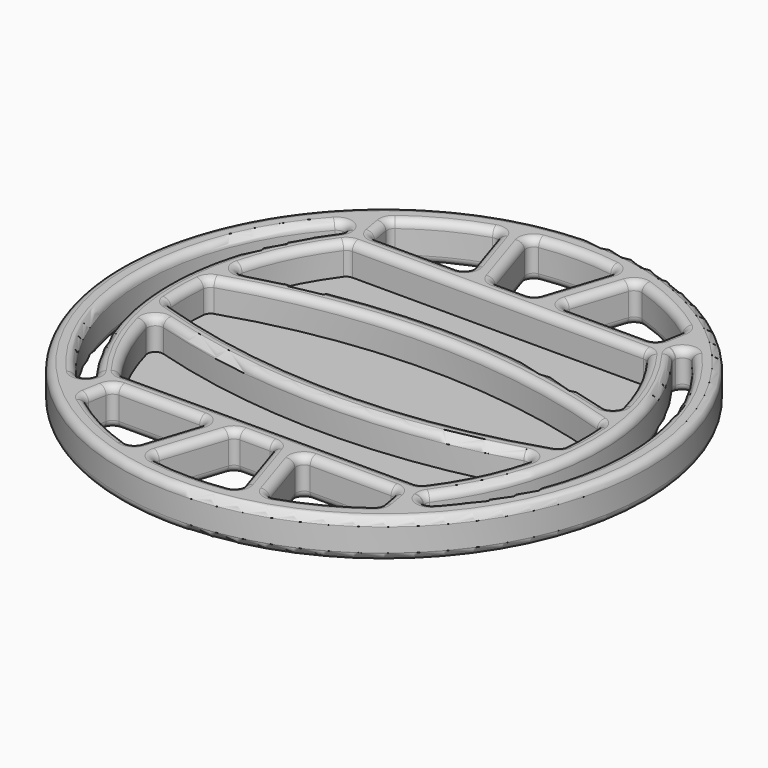
from build123d import *

# Parameters (mm, degrees)
F0_R     = 27.5
F1_DEPTH = 4
F2_DEPTH = 0.8
F3_F1_R  = 0.8
F3_F2_R  = 0.8
F3_F3_R  = 0.8


with BuildPart() as f1:
    # F0 (on Top) → F1 (new body)
    with BuildSketch(Plane.XY):
        Circle(F0_R)
        with BuildLine():
            ThreePointArc((17.4992602404, 17.994051546), (23.1218666205, 9.7667437759), (25.1, 0))
            ThreePointArc((25.1, 0), (23.1218666205, -9.7667437759), (17.4992602404, -17.994051546))
            ThreePointArc((17.4992602404, -17.994051546), (16.4683535979, -18.9421046818), (15.3861717662, -19.8311804586))
            ThreePointArc((15.3861717662, -19.8311804586), (11.4042701214, -22.359620368), (7.0196312763, -24.098439301))
            ThreePointArc((7.0196312763, -24.098439301), (5.8558617583, -24.4073530533), (4.6786166552, -24.6601002876))
            ThreePointArc((4.6786166552, -24.6601002876), (0, -25.1), (-4.6786166552, -24.6601002876))
            ThreePointArc((-4.6786166552, -24.6601002876), (-5.8558617583, -24.4073530533), (-7.0196312763, -24.098439301))
            ThreePointArc((-7.0196312763, -24.098439301), (-11.4042701214, -22.359620368), (-15.3861717662, -19.8311804586))
            ThreePointArc((-15.3861717662, -19.8311804586), (-16.4683535979, -18.9421046818), (-17.4992602404, -17.994051546))
            ThreePointArc((-17.4992602404, -17.994051546), (-25.1, 0), (-17.4992602404, 17.994051546))
            ThreePointArc((-17.4992602404, 17.994051546), (-16.4683535979, 18.9421046818), (-15.3861717662, 19.8311804586))
            ThreePointArc((-15.3861717662, 19.8311804586), (-11.4042701214, 22.359620368), (-7.0196312763, 24.098439301))
            ThreePointArc((-7.0196312763, 24.098439301), (-5.8558617583, 24.4073530533), (-4.6786166552, 24.6601002876))
            ThreePointArc((-4.6786166552, 24.6601002876), (0, 25.1), (4.6786166552, 24.6601002876))
            ThreePointArc((4.6786166552, 24.6601002876), (5.8558617583, 24.4073530533), (7.0196312763, 24.098439301))
            ThreePointArc((7.0196312763, 24.098439301), (11.4042701214, 22.359620368), (15.3861717662, 19.8311804586))
            ThreePointArc((15.3861717662, 19.8311804586), (16.4683535979, 18.9421046818), (17.4992602404, 17.994051546))
        make_face(mode=Mode.SUBTRACT)
        with BuildLine():
            Line((17.1548605167, 16.0408636544), (17.4992602404, 17.994051546))
            ThreePointArc((17.4992602404, 17.994051546), (16.4683535979, 18.9421046818), (15.3861717662, 19.8311804586))
            Line((15.3861717662, 19.8311804586), (14.8558084801, 16.8233407964))
            Line((14.8558084801, 16.8233407964), (4.6558084801, 16.8233407964))
            Line((4.6558084801, 16.8233407964), (2.1322991419, 16.8233407964))
            Line((2.1322991419, 16.8233407964), (0, 16.8233407964))
            Line((0, 16.8233407964), (-2.1322991419, 16.8233407964))
            Line((-2.1322991419, 16.8233407964), (-4.6558084801, 16.8233407964))
            Line((-4.6558084801, 16.8233407964), (-14.8558084801, 16.8233407964))
            Line((-14.8558084801, 16.8233407964), (-15.3861717662, 19.8311804586))
            ThreePointArc((-15.3861717662, 19.8311804586), (-16.4683535979, 18.9421046818), (-17.4992602404, 17.994051546))
            Line((-17.4992602404, 17.994051546), (-17.1548605167, 16.0408636544))
            ThreePointArc((-17.1548605167, 16.0408636544), (-22.6, 0), (-17.1548605167, -16.0408636544))
            Line((-17.1548605167, -16.0408636544), (-17.4992602404, -17.994051546))
            ThreePointArc((-17.4992602404, -17.994051546), (-16.4683535979, -18.9421046818), (-15.3861717662, -19.8311804586))
            Line((-15.3861717662, -19.8311804586), (-14.8558084801, -16.8233407964))
            Line((-14.8558084801, -16.8233407964), (-4.6558084801, -16.8233407964))
            Line((-4.6558084801, -16.8233407964), (-2.1322991419, -16.8233407964))
            Line((-2.1322991419, -16.8233407964), (0, -16.8233407964))
            Line((0, -16.8233407964), (2.1322991419, -16.8233407964))
            Line((2.1322991419, -16.8233407964), (4.6558084801, -16.8233407964))
            Line((4.6558084801, -16.8233407964), (14.8558084801, -16.8233407964))
            Line((14.8558084801, -16.8233407964), (15.3861717662, -19.8311804586))
            ThreePointArc((15.3861717662, -19.8311804586), (16.4683535979, -18.9421046818), (17.4992602404, -17.994051546))
            Line((17.4992602404, -17.994051546), (17.1548605167, -16.0408636544))
            ThreePointArc((17.1548605167, -16.0408636544), (22.6, 0), (17.1548605167, 16.0408636544))
        make_face()
        with BuildLine():
            ThreePointArc((-20.1097129023, 4.861748679), (-18.4060459784, 10.1010953169), (-15.5681538361, 14.8233407964))
            Line((-15.5681538361, 14.8233407964), (15.5681538361, 14.8233407964))
            ThreePointArc((15.5681538361, 14.8233407964), (18.4060459784, 10.1010953169), (20.1097129023, 4.861748679))
            ThreePointArc((20.1097129023, 4.861748679), (20.3085337575, 3.7562552412), (20.4561618511, 2.6427690852))
            ThreePointArc((20.4561618511, 2.6427690852), (20.6, 0), (20.4561618511, -2.6427690852))
            ThreePointArc((20.4561618511, -2.6427690852), (20.3085337575, -3.7562552412), (20.1097129023, -4.861748679))
            ThreePointArc((20.1097129023, -4.861748679), (18.4060459784, -10.1010953169), (15.5681538361, -14.8233407964))
            Line((15.5681538361, -14.8233407964), (-15.5681538361, -14.8233407964))
            ThreePointArc((-15.5681538361, -14.8233407964), (-18.4060459784, -10.1010953169), (-20.1097129023, -4.861748679))
            ThreePointArc((-20.1097129023, -4.861748679), (-20.3085337575, -3.7562552412), (-20.4561618511, -2.6427690852))
            ThreePointArc((-20.4561618511, -2.6427690852), (-20.6, 0), (-20.4561618511, 2.6427690852))
            ThreePointArc((-20.4561618511, 2.6427690852), (-20.3085337575, 3.7562552412), (-20.1097129023, 4.861748679))
        make_face(mode=Mode.SUBTRACT)
        with BuildLine():
            ThreePointArc((20.1097129023, 4.861748679), (0, 8), (-20.1097129023, 4.861748679))
            ThreePointArc((-20.1097129023, 4.861748679), (-20.3085337575, 3.7562552412), (-20.4561618511, 2.6427690852))
            ThreePointArc((-20.4561618511, 2.6427690852), (0, 6), (20.4561618511, 2.6427690852))
            ThreePointArc((20.4561618511, 2.6427690852), (20.3085337575, 3.7562552412), (20.1097129023, 4.861748679))
        make_face()
        with BuildLine():
            ThreePointArc((20.4561618511, -2.6427690852), (0, -6), (-20.4561618511, -2.6427690852))
            ThreePointArc((-20.4561618511, -2.6427690852), (-20.3085337575, -3.7562552412), (-20.1097129023, -4.861748679))
            ThreePointArc((-20.1097129023, -4.861748679), (0, -8), (20.1097129023, -4.861748679))
            ThreePointArc((20.1097129023, -4.861748679), (20.3085337575, -3.7562552412), (20.4561618511, -2.6427690852))
        make_face()
        with BuildLine():
            Line((-2.1322991419, 16.8233407964), (-4.6786166552, 24.6601002876))
            ThreePointArc((-4.6786166552, 24.6601002876), (-5.8558617583, 24.4073530533), (-7.0196312763, 24.098439301))
            Line((-7.0196312763, 24.098439301), (-4.6558084801, 16.8233407964))
            Line((-4.6558084801, 16.8233407964), (-2.1322991419, 16.8233407964))
        make_face()
        with BuildLine():
            Line((4.6558084801, 16.8233407964), (7.0196312763, 24.098439301))
            ThreePointArc((7.0196312763, 24.098439301), (5.8558617583, 24.4073530533), (4.6786166552, 24.6601002876))
            Line((4.6786166552, 24.6601002876), (2.1322991419, 16.8233407964))
            Line((2.1322991419, 16.8233407964), (4.6558084801, 16.8233407964))
        make_face()
        with BuildLine():
            ThreePointArc((-7.0196312763, -24.098439301), (-5.8558617583, -24.4073530533), (-4.6786166552, -24.6601002876))
            Line((-4.6786166552, -24.6601002876), (-2.1322991419, -16.8233407964))
            Line((-2.1322991419, -16.8233407964), (-4.6558084801, -16.8233407964))
            Line((-4.6558084801, -16.8233407964), (-7.0196312763, -24.098439301))
        make_face()
        with BuildLine():
            ThreePointArc((4.6786166552, -24.6601002876), (5.8558617583, -24.4073530533), (7.0196312763, -24.098439301))
            Line((7.0196312763, -24.098439301), (4.6558084801, -16.8233407964))
            Line((4.6558084801, -16.8233407964), (2.1322991419, -16.8233407964))
            Line((2.1322991419, -16.8233407964), (4.6786166552, -24.6601002876))
        make_face()
    extrude(amount=F1_DEPTH)

    # F0 (on Top) → F2 (join)
    with BuildSketch(Plane.XY):
        with BuildLine():
            Line((15.5681538361, 14.8233407964), (-15.5681538361, 14.8233407964))
            ThreePointArc((-15.5681538361, 14.8233407964), (-18.4060459784, 10.1010953169), (-20.1097129023, 4.861748679))
            ThreePointArc((-20.1097129023, 4.861748679), (0, 8), (20.1097129023, 4.861748679))
            ThreePointArc((20.1097129023, 4.861748679), (18.4060459784, 10.1010953169), (15.5681538361, 14.8233407964))
        make_face()
        with BuildLine():
            ThreePointArc((20.4561618511, 2.6427690852), (0, 6), (-20.4561618511, 2.6427690852))
            ThreePointArc((-20.4561618511, 2.6427690852), (-20.6, 0), (-20.4561618511, -2.6427690852))
            ThreePointArc((-20.4561618511, -2.6427690852), (0, -6), (20.4561618511, -2.6427690852))
            ThreePointArc((20.4561618511, -2.6427690852), (20.6, 0), (20.4561618511, 2.6427690852))
        make_face()
        with BuildLine():
            ThreePointArc((20.1097129023, -4.861748679), (0, -8), (-20.1097129023, -4.861748679))
            ThreePointArc((-20.1097129023, -4.861748679), (-18.4060459784, -10.1010953169), (-15.5681538361, -14.8233407964))
            Line((-15.5681538361, -14.8233407964), (15.5681538361, -14.8233407964))
            ThreePointArc((15.5681538361, -14.8233407964), (18.4060459784, -10.1010953169), (20.1097129023, -4.861748679))
        make_face()
    extrude(amount=F2_DEPTH)

    # F3: fillet of radius 0.8 on 114 edges, made by hand

    # F3_f1
    f3_f1_edges = [f1.edges().sort_by_distance(p)[0] for p in [
        (-15.3861717662, 19.8311804586, 2),
        (-4.6786166552, 24.6601002876, 2),
        (7.0196312763, 24.098439301, 2),
        (17.4992602404, 17.994051546, 2),
        (17.1548605167, 16.0408636544, 2),
        (17.1548605167, -16.0408636544, 2),
        (17.4992602404, -17.994051546, 2),
        (15.3861717662, 19.8311804586, 2),
        (14.8558084801, 16.8233407964, 2),
        (4.6558084801, 16.8233407964, 2),
        (4.6786166552, 24.6601002876, 2),
        (2.1322991419, 16.8233407964, 2),
        (-2.1322991419, 16.8233407964, 2),
        (-14.8558084801, 16.8233407964, 2),
        (-4.6558084801, 16.8233407964, 2),
        (-7.0196312763, 24.098439301, 2),
        (-17.4992602404, 17.994051546, 2),
        (-17.1548605167, 16.0408636544, 2),
        (-17.4992602404, -17.994051546, 2),
        (-17.1548605167, -16.0408636544, 2),
        (-15.5681538361, 14.8233407964, 2.4),
        (15.5681538361, 14.8233407964, 2.4),
        (20.1097129023, 4.861748679, 2.4),
        (-20.1097129023, 4.861748679, 2.4),
        (-20.4561618511, -2.6427690852, 2.4),
        (20.4561618511, -2.6427690852, 2.4),
        (20.4561618511, 2.6427690852, 2.4),
        (20.1097129023, -4.861748679, 2.4),
        (-20.1097129023, -4.861748679, 2.4),
        (-15.5681538361, -14.8233407964, 2.4),
        (15.5681538361, -14.8233407964, 2.4),
        (15.3861717662, -19.8311804586, 2),
        (14.8558084801, -16.8233407964, 2),
        (7.0196312763, -24.098439301, 2),
        (4.6558084801, -16.8233407964, 2),
        (4.6786166552, -24.6601002876, 2),
        (-4.6786166552, -24.6601002876, 2),
        (2.1322991419, -16.8233407964, 2),
        (-2.1322991419, -16.8233407964, 2),
        (-20.4561618511, 2.6427690852, 2.4),
        (-4.6558084801, -16.8233407964, 2),
        (-15.3861717662, -19.8311804586, 2),
        (-14.8558084801, -16.8233407964, 2),
        (-7.0196312763, -24.098439301, 2),
    ]]
    fillet(f3_f1_edges, radius=F3_F1_R)

    # F3_f2
    f3_f2_edges = [f1.edges().sort_by_distance(p)[0] for p in [
        (-27.5, 0, 0),
        (25.1, 0, 0),
        (-25.1, 0, 0),
        (-27.5, 0, 4),
        (-25.1, 0, 4),
        (25.1, 0, 4),
        (22.6, 0, 0),
        (-22.6, 0, 0),
        (22.6, 0, 4),
        (-22.6, 0, 4),
        (-17.2249911394, 16.0604439902, 4),
        (-17.2249911394, -16.0604439902, 4),
        (17.2249911394, -16.0604439902, 4),
        (17.2249911394, 16.0604439902, 4),
        (-17.2249911394, 16.0604439902, 0),
        (-17.2249911394, -16.0604439902, 0),
        (17.2249911394, -16.0604439902, 0),
        (17.2249911394, 16.0604439902, 0),
        (17.7928647513, 17.0773251864, 4),
        (17.7928647513, -17.0773251864, 4),
        (-17.7928647513, -17.0773251864, 4),
        (-17.7928647513, 17.0773251864, 4),
        (-17.7928647513, -17.0773251864, 0),
        (-17.7928647513, 17.0773251864, 0),
        (17.7928647513, 17.0773251864, 0),
        (17.7928647513, -17.0773251864, 0),
    ]]
    fillet(f3_f2_edges, radius=F3_F2_R)

    # F3_f3
    f3_f3_edges = [f1.edges().sort_by_distance(p)[0] for p in [
        (-9.9707213958, -16.8233407964, 0),
        (9.9707213958, -16.8233407964, 0),
        (-9.9707213958, 16.8233407964, 0),
        (9.9707213958, 16.8233407964, 0),
        (-9.9707213958, 16.8233407964, 4),
        (9.9707213958, 16.8233407964, 4),
        (0, 8, 4),
        (0, -6, 4),
        (0, -14.8233407964, 4),
        (9.9707213958, -16.8233407964, 4),
        (-9.9707213958, -16.8233407964, 4),
        (15.1369126796, -18.4175619328, 0),
        (15.1369126796, -18.4175619328, 4),
        (11.5400061519, -22.2898689546, 0),
        (11.5400061519, -22.2898689546, 4),
        (5.8860694276, -20.609694661, 0),
        (0, -25.1, 0),
        (-3.3522598692, -20.5779938427, 0),
        (0, -16.8233407964, 0),
        (3.3522598692, -20.5779938427, 0),
        (-11.5400061519, -22.2898689546, 0),
        (-15.1369126796, -18.4175619328, 0),
        (-5.8860694276, -20.609694661, 0),
        (15.1369126796, 18.4175619328, 0),
        (5.8860694276, 20.609694661, 0),
        (11.5400061519, 22.2898689546, 0),
        (0, 16.8233407964, 0),
        (-3.3522598692, 20.5779938427, 0),
        (0, 25.1, 0),
        (3.3522598692, 20.5779938427, 0),
        (-15.1369126796, 18.4175619328, 0),
        (-11.5400061519, 22.2898689546, 0),
        (-5.8860694276, 20.609694661, 0),
        (5.8860694276, -20.609694661, 4),
        (0, -25.1, 4),
        (-3.3522598692, -20.5779938427, 4),
        (0, -16.8233407964, 4),
        (3.3522598692, -20.5779938427, 4),
        (-11.5400061519, -22.2898689546, 4),
        (-15.1369126796, -18.4175619328, 4),
        (-5.8860694276, -20.609694661, 4),
        (15.1369126796, 18.4175619328, 4),
        (5.8860694276, 20.609694661, 4),
        (11.5400061519, 22.2898689546, 4),
        (0, 16.8233407964, 4),
        (-3.3522598692, 20.5779938427, 4),
        (0, 25.1, 4),
        (3.3522598692, 20.5779938427, 4),
        (-15.1369126796, 18.4175619328, 4),
        (-11.5400061519, 22.2898689546, 4),
        (-5.8860694276, 20.609694661, 4),
        (-18.191241448, -10.5595655082, 4),
        (0, -8, 4),
        (18.191241448, -10.5595655082, 4),
        (-20.6, 0, 4),
        (0, 6, 4),
        (20.6, 0, 4),
        (-18.191241448, 10.5595655082, 4),
        (0, 14.8233407964, 4),
        (18.191241448, 10.5595655082, 4),
        (15.5293152775, 14.7378691044, 4),
        (19.5703685704, 5.4631188781, 4),
        (-15.5293152775, 14.7378691044, 4),
        (-19.570368571, 5.4631188784, 4),
        (20.3376947293, 2.5446852874, 4),
        (20.3376947293, -2.5446852874, 4),
        (-20.3376947293, 2.5446852874, 4),
        (-20.3376947293, -2.5446852874, 4),
        (19.5703685704, -5.4631188781, 4),
        (15.5293152775, -14.7378691044, 4),
        (-19.5703685704, -5.4631188781, 4),
        (-15.5293152775, -14.7378691044, 4),
        (-7.1741517695, 23.8146449293, 4),
        (-5.1097004209, 17.1531125945, 4),
        (-15.2571022794, 19.7849345203, 4),
        (-14.6987588629, 17.0105052419, 4),
        (4.3123960679, 24.4474789452, 4),
        (2.0212933213, 16.9761272009, 4),
        (-4.3123960679, 24.4474789452, 4),
        (-2.0212933213, 16.9761272009, 4),
        (7.1741517695, 23.8146449293, 4),
        (15.2571022794, 19.7849345203, 4),
        (5.1097004209, 17.1531125945, 4),
        (14.6987588629, 17.0105052419, 4),
        (-5.1097004209, -17.1531125945, 4),
        (-7.1741517695, -23.8146449293, 4),
        (-15.2571022794, -19.7849345203, 4),
        (-14.6987588629, -17.0105052419, 4),
        (2.0212933213, -16.9761272009, 4),
        (4.3123960679, -24.4474789452, 4),
        (-2.0212933213, -16.9761272009, 4),
        (-4.3123960679, -24.4474789452, 4),
        (7.1741517695, -23.8146449293, 4),
        (5.1097004209, -17.1531125945, 4),
        (-7.1741517695, 23.8146449293, 0),
        (-5.1097004209, 17.1531125945, 0),
        (-15.2571022794, 19.7849345203, 0),
        (-14.6987588629, 17.0105052419, 0),
        (4.3123960679, 24.4474789452, 0),
        (2.0212933213, 16.9761272009, 0),
        (-4.3123960679, 24.4474789452, 0),
        (-2.0212933213, 16.9761272009, 0),
        (7.1741517695, 23.8146449293, 0),
        (15.2571022794, 19.7849345203, 0),
        (5.1097004209, 17.1531125945, 0),
        (14.6987588629, 17.0105052419, 0),
        (-5.1097004209, -17.1531125945, 0),
        (-7.1741517695, -23.8146449293, 0),
        (-15.2571022794, -19.7849345203, 0),
        (-14.6987588629, -17.0105052419, 0),
        (2.0212933213, -16.9761272009, 0),
        (4.3123960679, -24.4474789452, 0),
        (-2.0212933213, -16.9761272009, 0),
        (-4.3123960679, -24.4474789452, 0),
        (7.1741517695, -23.8146449293, 0),
        (5.1097004209, -17.1531125945, 0),
        (15.2571022794, -19.7849345203, 4),
        (15.2571022794, -19.7849345203, 0),
        (14.6987588629, -17.0105052419, 4),
        (14.6987588629, -17.0105052419, 0),
    ]]
    fillet(f3_f3_edges, radius=F3_F3_R)


solid = f1.part
